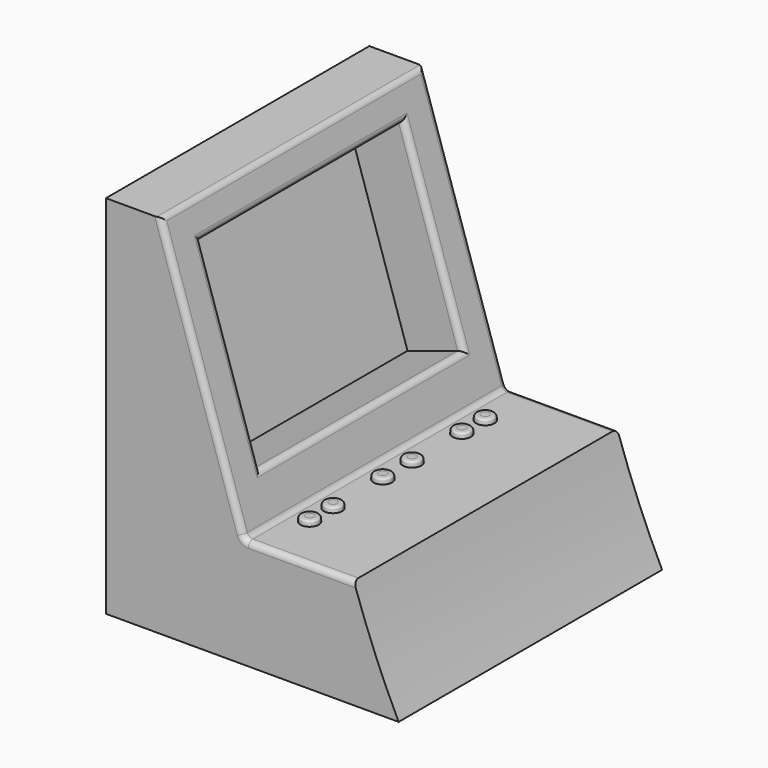
from build123d import *

# Parameters (mm, degrees)
F1_DEPTH = 450
F2_W     = 347
F2_H     = 261
F3_DEPTH = 80
F4_F1_R  = 8
F4_F2_R  = 8
F5_R     = 12.5
F6_DEPTH = 7


# Not quite as in the source:
# - a fillet or chamfer that OpenCascade refuses, or shapes differently, is made with other operations: its cross-section is extruded or revolved along the edge and cut away or added


with BuildPart() as f1:
    # F0 (on Front) → F1 (new body)
    with BuildSketch(Plane.XZ):
        with BuildLine():
            Line((-120.4737946391, 342.6808416843), (-195.4737946391, 342.6808416843))
            Line((-195.4737946391, 342.6808416843), (-195.4737946391, -157.3191583157))
            Line((-195.4737946391, -157.3191583157), (204.5262053609, -157.3191583157))
            ThreePointArc((204.5262053609, -157.3191583157), (171.3461744918, -83.3583725961), (143.2543578127, -7.3191583157))
            Line((143.2543578127, -7.3191583157), (-6.7456421873, -7.3191583157))
            Line((-6.7456421873, -7.3191583157), (-120.4737946391, 342.6808416843))
        make_face()
    extrude(amount=F1_DEPTH)

    # F2 (on face) → F3 (cut)
    with BuildSketch(Plane(origin=(-8.2525689762, 0, -2.681569779), x_dir=(0, 1, 0), z_dir=(0.951051518, 0, 0.3090323772))):
        with Locations((-225, 188.1374378125)):
            Rectangle(F2_W, F2_H)
    extrude(amount=-F3_DEPTH, mode=Mode.SUBTRACT)

    # F4: fillet of radius 8 on 8 edges, made by hand

    # F4_f1
    f4_f1_edges = [f1.edges().sort_by_distance(p)[0] for p in [
        (-6.7456421873, -225, -7.3191583157),
    ]]
    fillet(f4_f1_edges, radius=F4_F1_R)

    # F4_f2
    f4_f2_edges = [f1.edges().sort_by_distance(p)[0] for p in [
        (-64.5078037977, 0, 170.4447121755),
        (-64.5078037977, -450, 170.4447121755),
        (-120.4737946391, -225, 342.6808416843),
        (-66.3931286265, -398.5, 176.2468260396),
        (-106.7218538531, -225, 300.3590491347),
        (-66.3931286265, -51.5, 176.2468260396),
        (-26.0644034, -225, 52.1346029445),
        (-5.6356304889, -450, -5.791332299),
        (-5.6356304889, 0, -5.791332299),
    ]]
    fillet(f4_f2_edges, radius=F4_F2_R)

    # F5 (on face) → F6 (join)
    with BuildSketch(Plane.XY.offset(-7.3191583157)):
        with Locations((20.8874940872, -372.5)):
            Circle(F5_R)
        with Locations((20.8874940872, -332.5)):
            Circle(F5_R)
        with Locations((20.8874940872, -247.5)):
            Circle(F5_R)
        with Locations((20.8874940872, -197.5)):
            Circle(F5_R)
        with Locations((20.8874940872, -112.5)):
            Circle(F5_R)
        with Locations((20.8874940872, -72.5)):
            Circle(F5_R)
    extrude(amount=F6_DEPTH)

    # F7: fillet of radius 7 on 1 edges, made by hand

    # F7_s1 → F7_t2 (revolve, cut)
    with BuildSketch(Plane.XZ.offset(372.5)):
        with BuildLine():
            add(Edge.make_bspline(
                [(33.3874940872, -7.3191583157), (33.3874940872, -0.3191583157), (26.3874940872, -0.3191583157)],
                knots=[0, 0, 0, 1, 1, 1], degree=2, weights=[1, 2.3333333333, 1]))
            Line((26.3874940872, -0.3191583157), (33.3874940872, -0.3191583157))
            Line((33.3874940872, -0.3191583157), (33.3874940872, -7.3191583157))
        make_face()
    revolve(axis=Axis((20.8874940872, -372.5, -0.3191583157), (0, 0, 1)), mode=Mode.SUBTRACT)

    # F8: fillet of radius 7 on 5 edges, made by hand

    # F8_s1 → F8_t2 (revolve, cut)
    with BuildSketch(Plane.XZ.offset(332.5)):
        with BuildLine():
            add(Edge.make_bspline(
                [(33.3874940872, -7.3191583157), (33.3874940872, -0.3191583157), (26.3874940872, -0.3191583157)],
                knots=[0, 0, 0, 1, 1, 1], degree=2, weights=[1, 2.3333333333, 1]))
            Line((26.3874940872, -0.3191583157), (33.3874940872, -0.3191583157))
            Line((33.3874940872, -0.3191583157), (33.3874940872, -7.3191583157))
        make_face()
    revolve(axis=Axis((20.8874940872, -332.5, -0.3191583157), (0, 0, 1)), mode=Mode.SUBTRACT)

    # F8_s3 → F8_t4 (revolve, cut)
    with BuildSketch(Plane.XZ.offset(197.5)):
        with BuildLine():
            add(Edge.make_bspline(
                [(33.3874940872, -7.3191583157), (33.3874940872, -0.3191583157), (26.3874940872, -0.3191583157)],
                knots=[0, 0, 0, 1, 1, 1], degree=2, weights=[1, 2.3333333333, 1]))
            Line((26.3874940872, -0.3191583157), (33.3874940872, -0.3191583157))
            Line((33.3874940872, -0.3191583157), (33.3874940872, -7.3191583157))
        make_face()
    revolve(axis=Axis((20.8874940872, -197.5, -0.3191583157), (0, 0, 1)), mode=Mode.SUBTRACT)

    # F8_s5 → F8_t6 (revolve, cut)
    with BuildSketch(Plane.XZ.offset(247.5)):
        with BuildLine():
            add(Edge.make_bspline(
                [(33.3874940872, -7.3191583157), (33.3874940872, -0.3191583157), (26.3874940872, -0.3191583157)],
                knots=[0, 0, 0, 1, 1, 1], degree=2, weights=[1, 2.3333333333, 1]))
            Line((26.3874940872, -0.3191583157), (33.3874940872, -0.3191583157))
            Line((33.3874940872, -0.3191583157), (33.3874940872, -7.3191583157))
        make_face()
    revolve(axis=Axis((20.8874940872, -247.5, -0.3191583157), (0, 0, 1)), mode=Mode.SUBTRACT)

    # F8_s7 → F8_t8 (revolve, cut)
    with BuildSketch(Plane.XZ.offset(112.5)):
        with BuildLine():
            add(Edge.make_bspline(
                [(33.3874940872, -7.3191583157), (33.3874940872, -0.3191583157), (26.3874940872, -0.3191583157)],
                knots=[0, 0, 0, 1, 1, 1], degree=2, weights=[1, 2.3333333333, 1]))
            Line((26.3874940872, -0.3191583157), (33.3874940872, -0.3191583157))
            Line((33.3874940872, -0.3191583157), (33.3874940872, -7.3191583157))
        make_face()
    revolve(axis=Axis((20.8874940872, -112.5, -0.3191583157), (0, 0, 1)), mode=Mode.SUBTRACT)

    # F8_s9 → F8_t10 (revolve, cut)
    with BuildSketch(Plane.XZ.offset(72.5)):
        with BuildLine():
            add(Edge.make_bspline(
                [(33.3874940872, -7.3191583157), (33.3874940872, -0.3191583157), (26.3874940872, -0.3191583157)],
                knots=[0, 0, 0, 1, 1, 1], degree=2, weights=[1, 2.3333333333, 1]))
            Line((26.3874940872, -0.3191583157), (33.3874940872, -0.3191583157))
            Line((33.3874940872, -0.3191583157), (33.3874940872, -7.3191583157))
        make_face()
    revolve(axis=Axis((20.8874940872, -72.5, -0.3191583157), (0, 0, 1)), mode=Mode.SUBTRACT)


solid = f1.part
